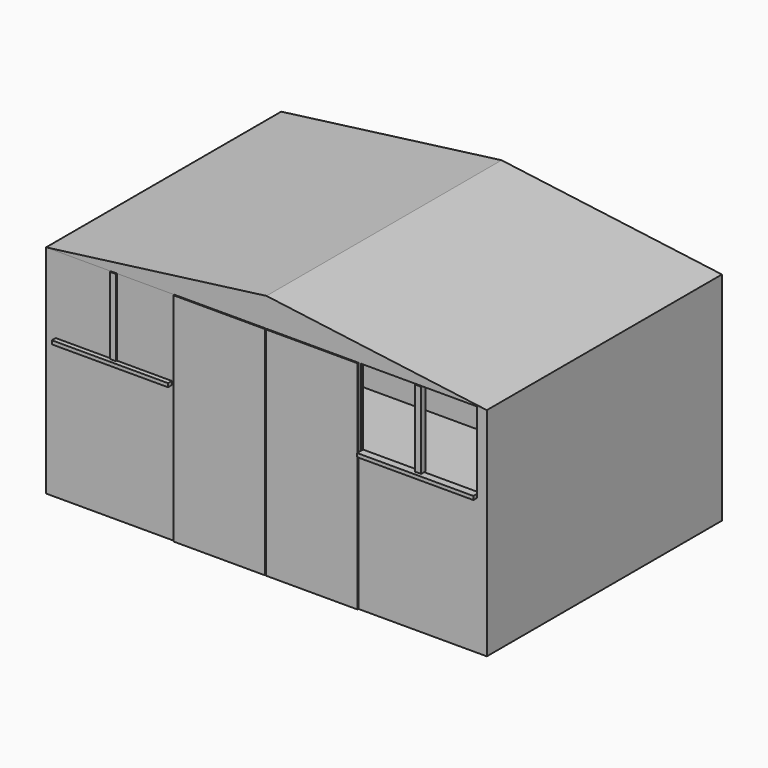
from build123d import *

# Parameters (mm, degrees)
F0_W          = 366
F0_H          = 244
F0_W_2        = 361.6
F0_H_2        = 239.6
F1_DEPTH      = 180
F2_DEPTH      = 2.2
F3_W          = 76
F3_H          = 180
F3_W_2        = 5
F3_H_2        = 63.7124854326
F4_DEPTH      = 1
F4_DEPTH_BACK = 3.3
F3_W_3        = 45.75
F5_DEPTH      = 25
F6_DEPTH      = 8
F7_DEPTH      = 4
F9_DEPTH      = 244


# Not quite as in the source:
# - a feature names something its author has since deleted; it is built from what else it names


with BuildPart() as f1:
    # F0 (on Top) → F1 (new body)
    with BuildSketch(Plane.XY):
        with Locations((183, -122)):
            Rectangle(F0_W, F0_H)
        with Locations((183, -122)):
            Rectangle(F0_W_2, F0_H_2, mode=Mode.SUBTRACT)
    extrude(amount=F1_DEPTH)

    # F0 (on Top) → F2 (join)
    with BuildSketch(Plane.XY):
        with Locations((183, -122)):
            Rectangle(F0_W_2, F0_H_2)
    extrude(amount=F2_DEPTH)

    # F3 (on face) → F4 (join, two sides)
    with BuildSketch(Plane.XZ.offset(244)) as f4_sk:
        with Locations((144.5, 90)):
            Rectangle(F3_W, F3_H)
        with Locations((221.5, 90)):
            Rectangle(F3_W, F3_H)
        with Locations((56.25, 148.1437572837)):
            Rectangle(F3_W_2, F3_H_2)
        with Locations((309.75, 148.1437572837)):
            Rectangle(F3_W_2, F3_H_2)
    extrude(amount=F4_DEPTH)
    extrude(f4_sk.sketch, amount=-F4_DEPTH_BACK)

    # F3 (on face) → F5 (cut)
    with BuildSketch(Plane.XZ.offset(244)):
        Polygon((104.5, 180), (106.5, 180), (182.5, 180), (183.5, 180), (259.5, 180), (261.5, 180), (307.25, 180), (312.25, 180), (358, 180), (366, 180), (183, 204), (0, 180), (8, 180), (53.75, 180), (58.75, 180), align=None)
        with Locations((284.375, 148.1437572837)):
            Rectangle(F3_W_3, F3_H_2)
        with Locations((335.125, 148.1437572837)):
            Rectangle(F3_W_3, F3_H_2)
    extrude(amount=-F5_DEPTH, mode=Mode.SUBTRACT)

    # F3 (on face) → F6 (join)
    with BuildSketch(Plane.XZ.offset(244)):
        Polygon((104.5, 180), (106.5, 180), (182.5, 180), (183.5, 180), (259.5, 180), (261.5, 180), (307.25, 180), (312.25, 180), (358, 180), (366, 180), (183, 204), (0, 180), (8, 180), (53.75, 180), (58.75, 180), align=None)
    extrude(amount=-F6_DEPTH)

    # F3 (on face) → F7 (join)
    with BuildSketch(Plane.XZ.offset(244)):
        Polygon((307.25, 116.2875145674), (261.5, 116.2875145674), (261.5, 113.2875145674), (358, 113.2875145674), (358, 116.2875145674), (312.25, 116.2875145674), align=None)
        Polygon((104.5, 113.2875145674), (104.5, 116.2875145674), (58.75, 116.2875145674), (53.75, 116.2875145674), (8, 116.2875145674), (8, 113.2875145674), align=None)
    extrude(amount=F7_DEPTH)


with BuildPart() as f9:
    # F8 (on face) → F9 (new body)
    with BuildSketch(Plane(origin=(0, 0, 0), x_dir=(-1, 0, 0), z_dir=(0, 1, 0))):
        Polygon((-183, 204), (-366, 180), (0, 180), align=None)
    extrude(amount=-F9_DEPTH)


solid = Compound([f1.part, f9.part])
